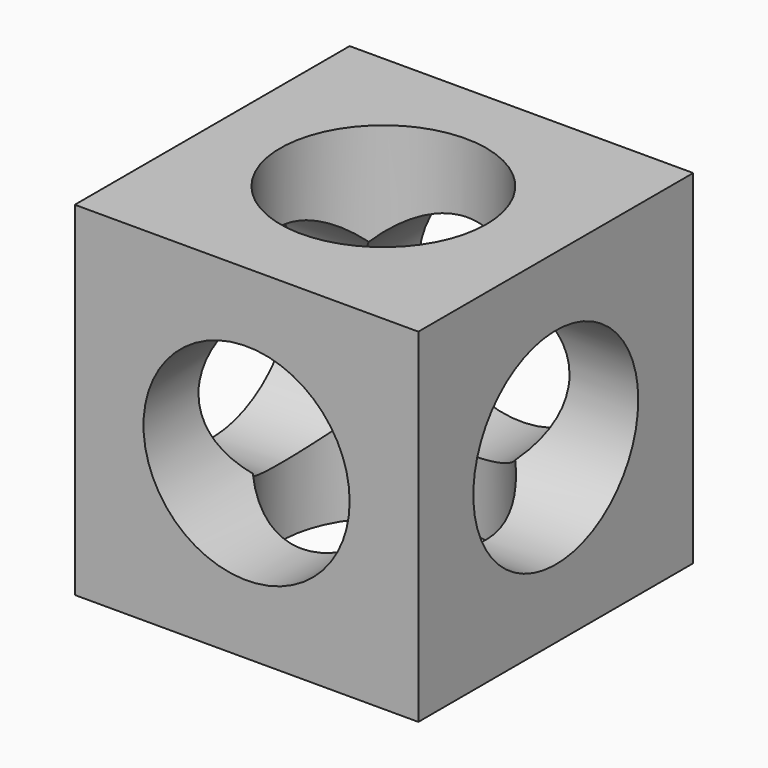
from build123d import *
from build123d import SkipClean  # not in build123d's __all__

# Parameters (mm, degrees)
F0_W      = 127
F0_H      = 127
F1_DEPTH  = 127
F2_R      = 38.1
F3_DEPTH  = 76.2
F4_R      = 38.1
F6_DEPTH  = 76.2
F7_R      = 38.1
F9_DEPTH  = 76.2
F10_R     = 38.1
F11_DEPTH = 76.2
F12_R     = 38.1
F13_DEPTH = 76.2
F14_R     = 38.1
F15_DEPTH = 76.2


with BuildPart() as f1:
    # F0 (on Front) → F1 (new body)
    with BuildSketch(Plane.XZ):
        with Locations((63.5, 63.5)):
            Rectangle(F0_W, F0_H)
    extrude(amount=F1_DEPTH)

    # F2 (on face) → F3 (cut)
    with BuildSketch(Plane.XZ.offset(127)):
        with Locations((63.5, 63.5)):
            Circle(F2_R)
    extrude(amount=-F3_DEPTH, mode=Mode.SUBTRACT)

    # F4 (on face) → F6 (cut)
    with BuildSketch(Plane(origin=(0, 0, 0), x_dir=(0, -1, 0), z_dir=(-1, 0, 0))):
        with Locations((63.5, 63.5)):
            Circle(F4_R)
    extrude(amount=-F6_DEPTH, mode=Mode.SUBTRACT)

    # F7 (on face) → F9 (cut)
    with BuildSketch(Plane.YZ.offset(127)):
        with Locations((-63.5, 63.5)):
            Circle(F7_R)
    with SkipClean():  # cleaning this boolean's faces spoils the solid; the shape is the same uncleaned
        extrude(amount=-F9_DEPTH, mode=Mode.SUBTRACT)

    # F10 (on face) → F11 (cut)
    with BuildSketch(Plane(origin=(0, 0, 0), x_dir=(-1, 0, 0), z_dir=(0, 1, 0))):
        with Locations((-63.5, 63.5)):
            Circle(F10_R)
    extrude(amount=-F11_DEPTH, mode=Mode.SUBTRACT)

    # F12 (on face) → F13 (cut)
    with BuildSketch(Plane.XY.offset(127)):
        with Locations((62.3162926857, -62.3162926857)):
            Circle(F12_R)
    extrude(amount=-F13_DEPTH, mode=Mode.SUBTRACT)

    # F14 (on face) → F15 (cut)
    with BuildSketch(Plane(origin=(0, 0, 0), x_dir=(1, 0, 0), z_dir=(0, 0, -1))):
        with Locations((63.5, 63.5)):
            Circle(F14_R)
    extrude(amount=-F15_DEPTH, mode=Mode.SUBTRACT)


solid = f1.part
